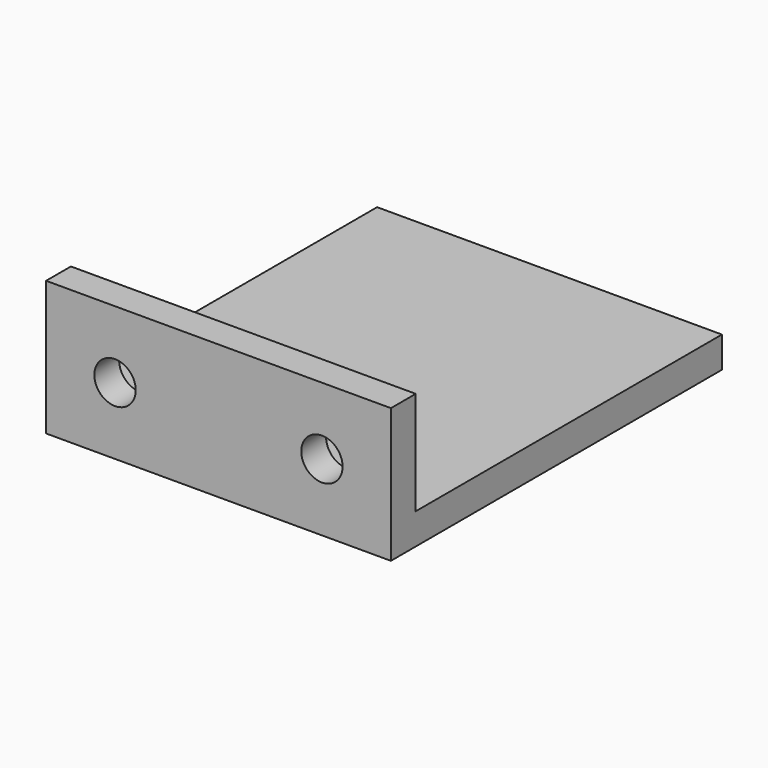
from build123d import *

# Parameters (mm, degrees)
F1_DEPTH = 100
F2_R     = 6
F3_DEPTH = 25


with BuildPart() as f1:
    # F0 (on Right) → F1 (new body)
    with BuildSketch(Plane.YZ):
        Polygon((9, 0), (0, 0), (0, -38.9847982002), (120, -38.9847982002), (120, -29.9847982002), (9, -29.9847982002), align=None)
    extrude(amount=F1_DEPTH)

    # F2 (on face) → F3 (cut)
    with BuildSketch(Plane.XZ):
        with Locations((20, -19.4923991001)):
            Circle(F2_R)
        with Locations((80, -19.4923991001)):
            Circle(F2_R)
    extrude(amount=-F3_DEPTH, mode=Mode.SUBTRACT)


solid = f1.part
